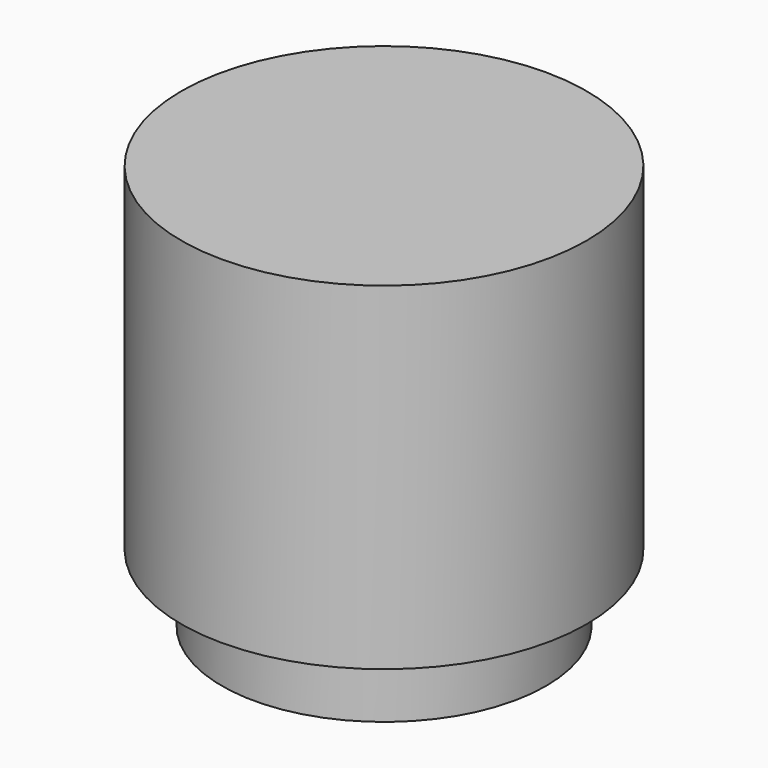
from build123d import *


# Not quite as in the source:
# - a feature names something its author has since deleted; it is built from what else it names


with BuildPart() as f1:
    # F0 (on Front) → F1 (revolve)
    with BuildSketch(Plane.XZ):
        with BuildLine():
            Line((-15, -25), (-12, -25))
            Line((-12, -25), (-12, -30))
            Line((-12, -30), (-9, -30))
            Line((-9, -30), (-9, -7.2415010072))
            ThreePointArc((-9, -7.2415010072), (-4.9914312836, -4.0779872119), (0, -3))
            Line((0, -3), (0, 0))
            Line((0, 0), (-15, 0))
            Line((-15, 0), (-15, -3))
            Line((-15, -3), (-15, -25))
        make_face()
    revolve(axis=Axis((0, 0, -1.5), (0, 0, -1)))


solid = f1.part
